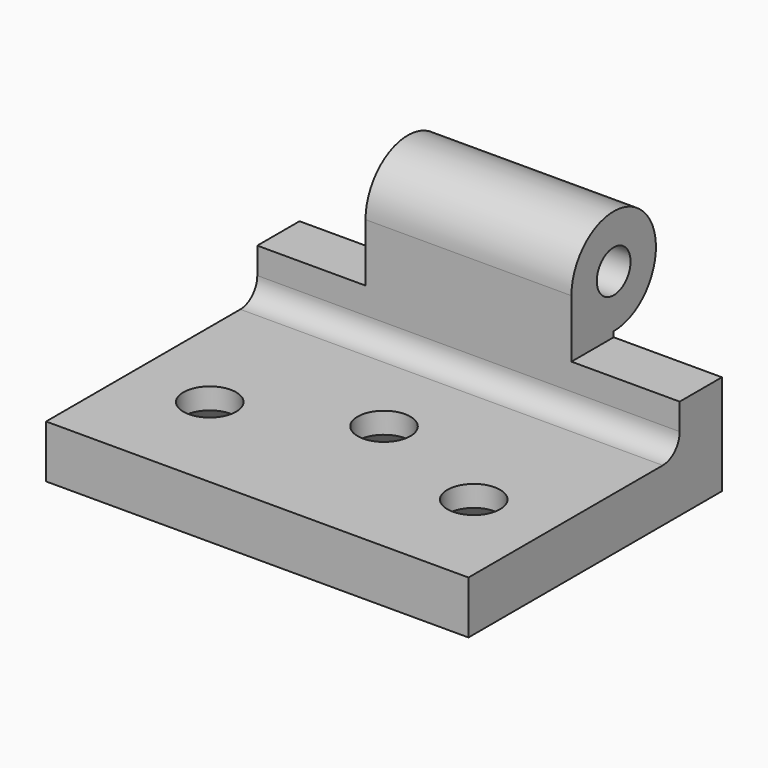
from build123d import *

# Parameters (mm, degrees)
F0_R           = 2
F1_DEPTH       = 20
F3_W           = 10.25
F3_H           = 12
F4_DEPTH       = 10.501
F5_R           = 2
F7_D           = 5
F7_CSINK_D     = 11
F7_CSINK_ANGLE = 90


# Not quite as in the source:
# - a pattern or mirror of a feature is missing from the dataset's text; its kind, count and spacing are read off the source's solid


with BuildPart() as f1:
    # F0 (on Right) → F1 (new body, symmetric)
    with BuildSketch(Plane.YZ):
        with BuildLine():
            Line((0, 5), (0, 0))
            Line((0, 0), (30, 0))
            Line((30, 0), (30, 10))
            ThreePointArc((30, 10), (33.5355339059, 18.5355339059), (25, 15))
            Line((25, 15), (25, 5))
            Line((25, 5), (0, 5))
        make_face()
        with Locations((30, 15)):
            Circle(F0_R, mode=Mode.SUBTRACT)
    extrude(amount=F1_DEPTH, both=True)

    # F3 (on offset) → F4 (cut, through all)
    with BuildSketch(Plane.XY.offset(9.5)):
        with Locations((14.875, 31)):
            Rectangle(F3_W, F3_H)
    f4 = extrude(amount=F4_DEPTH, mode=Mode.SUBTRACT)

    # F4_copies: F4 across plane
    add(f4.mirror(Plane(origin=(0, 0, 0), x_dir=(0, 0, -1), z_dir=(-1, 0, 0))), mode=Mode.SUBTRACT)

    # F5
    f5_edges = [f1.edges().sort_by_distance(p)[0] for p in [
        (0, 25, 5),
    ]]
    fillet(f5_edges, radius=F5_R)

    # F7 (through all)
    with Locations(Plane(origin=(0, 0, 0), x_dir=(1, 0, 0), z_dir=(0, 0, -1))):
        with Locations((-12.5, -10), (0, -15), (12.5, -10)):
            CounterSinkHole(F7_D / 2, F7_CSINK_D / 2, counter_sink_angle=F7_CSINK_ANGLE)


solid = f1.part
